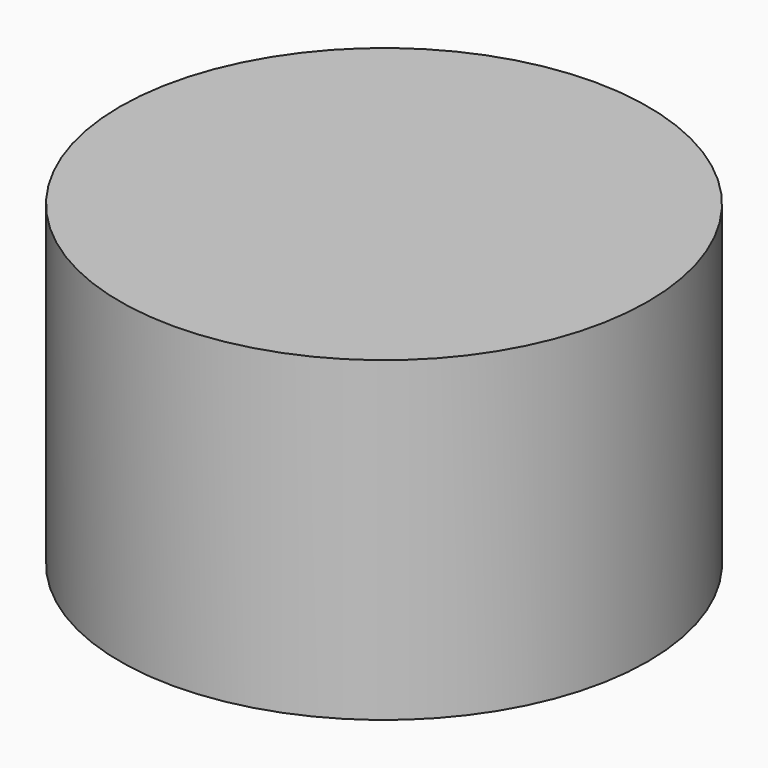
from build123d import *

# Parameters (mm, degrees)
F0_R     = 31.75
F1_DEPTH = 38.1


# Not quite as in the source:
# - a feature of the source that left no trace in its solid (it failed there, or was rolled back) is left out


with BuildPart() as f1:
    # F0 (on Top) → F1 (new body)
    with BuildSketch(Plane.XY):
        Circle(F0_R)
    extrude(amount=F1_DEPTH)


solid = f1.part
